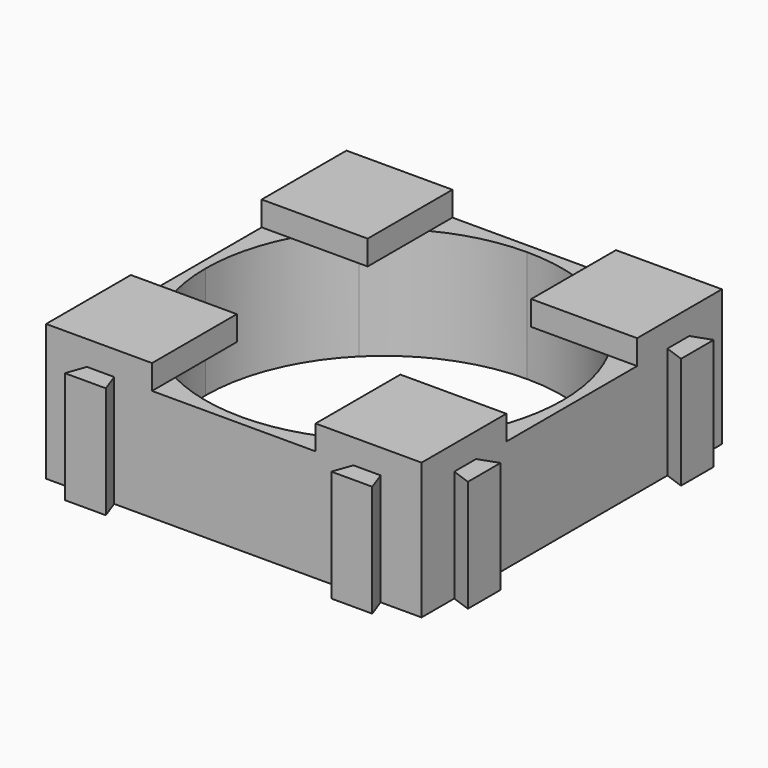
from build123d import *

# Parameters (mm, degrees)
F1_DEPTH = 8.2
F2_W     = 7.775
F2_H     = 7.775
F3_DEPTH = 1.8


# Not quite as in the source:
# - a feature names something its author has since deleted; it is built from what else it names


with BuildPart() as f1:
    # F0 (on Top) → F1 (new body)
    with BuildSketch(Plane.XY):
        with BuildLine():
            Line((13.775, 10.775), (13.775, 13.775))
            Line((13.775, 13.775), (10.775, 13.775))
            Line((10.775, 13.775), (11.275, 12.375))
            Line((11.275, 12.375), (8.275, 12.375))
            Line((8.275, 12.375), (8.775, 13.775))
            Line((8.775, 13.775), (0, 13.775))
            Line((0, 13.775), (0, 13.1))
            ThreePointArc((0, 13.1), (9.2630988335, 9.2630988335), (13.1, 0))
            Line((13.1, 0), (13.775, 0))
            Line((13.775, 0), (13.775, 8.775))
            Line((13.775, 8.775), (13.775, 10.775))
        make_face()
        Polygon((15.175, 11.275), (13.775, 10.775), (13.775, 8.775), (15.175, 8.275), align=None)
        Polygon((15.175, -8.275), (13.775, -8.775), (13.775, -10.775), (15.175, -11.275), align=None)
        with BuildLine():
            Line((13.775, -8.775), (13.775, 0))
            Line((13.775, 0), (13.1, 0))
            ThreePointArc((13.1, 0), (12.1028218759, -5.013152964), (9.2630988335, -9.2630988335))
            Line((9.2630988335, -9.2630988335), (13.775, -13.775))
            Line((13.775, -13.775), (13.775, -10.775))
            Line((13.775, -10.775), (13.775, -8.775))
        make_face()
        with BuildLine():
            Line((13.775, -13.775), (9.2630988335, -9.2630988335))
            ThreePointArc((9.2630988335, -9.2630988335), (5.013152964, -12.1028218759), (0, -13.1))
            Line((0, -13.1), (0, -13.775))
            Line((0, -13.775), (8.775, -13.775))
            Line((8.775, -13.775), (10.775, -13.775))
            Line((10.775, -13.775), (13.775, -13.775))
        make_face()
        Polygon((11.275, -15.175), (10.775, -13.775), (8.775, -13.775), (8.275, -15.175), align=None)
        with BuildLine():
            ThreePointArc((0, -13.1), (-9.2630988335, -9.2630988335), (-13.1, 0))
            Line((-13.1, 0), (-13.775, 0))
            Line((-13.775, 0), (-13.775, -8.775))
            Line((-13.775, -8.775), (-12.375, -8.275))
            Line((-12.375, -8.275), (-12.375, -11.275))
            Line((-12.375, -11.275), (-13.775, -10.775))
            Line((-13.775, -10.775), (-13.775, -13.775))
            Line((-13.775, -13.775), (-10.775, -13.775))
            Line((-10.775, -13.775), (-8.775, -13.775))
            Line((-8.775, -13.775), (0, -13.775))
            Line((0, -13.775), (0, -13.1))
        make_face()
        Polygon((-8.275, -15.175), (-8.775, -13.775), (-10.775, -13.775), (-11.275, -15.175), align=None)
        with BuildLine():
            ThreePointArc((-13.1, 0), (-12.1028218759, 5.013152964), (-9.2630988335, 9.2630988335))
            Line((-9.2630988335, 9.2630988335), (-13.775, 13.775))
            Line((-13.775, 13.775), (-13.775, 10.775))
            Line((-13.775, 10.775), (-12.375, 11.275))
            Line((-12.375, 11.275), (-12.375, 8.275))
            Line((-12.375, 8.275), (-13.775, 8.775))
            Line((-13.775, 8.775), (-13.775, 0))
            Line((-13.775, 0), (-13.1, 0))
        make_face()
        with BuildLine():
            Line((0, 13.1), (0, 13.775))
            Line((0, 13.775), (-8.775, 13.775))
            Line((-8.775, 13.775), (-8.275, 12.375))
            Line((-8.275, 12.375), (-9.775, 12.375))
            Line((-9.775, 12.375), (-11.275, 12.375))
            Line((-11.275, 12.375), (-10.775, 13.775))
            Line((-10.775, 13.775), (-13.775, 13.775))
            Line((-13.775, 13.775), (-9.2630988335, 9.2630988335))
            ThreePointArc((-9.2630988335, 9.2630988335), (-5.013152964, 12.1028218759), (0, 13.1))
        make_face()
    extrude(amount=F1_DEPTH)

    # F2 (on face) → F3 (join)
    with BuildSketch(Plane.XY.offset(8.2)):
        Polygon((-6, 13.775), (-13.775, 13.775), (-6, 6), align=None)
        Polygon((-6, -13.775), (-6, -6), (-13.775, -13.775), align=None)
        Polygon((-13.775, -13.775), (-6, -6), (-13.775, -6), align=None)
        Polygon((-6, 6), (-13.775, 13.775), (-13.775, 6), align=None)
        with Locations((9.8875, -9.8875)):
            Rectangle(F2_W, F2_H)
        with Locations((9.8875, 9.8875)):
            Rectangle(F2_W, F2_H)
    extrude(amount=F3_DEPTH)


solid = f1.part
